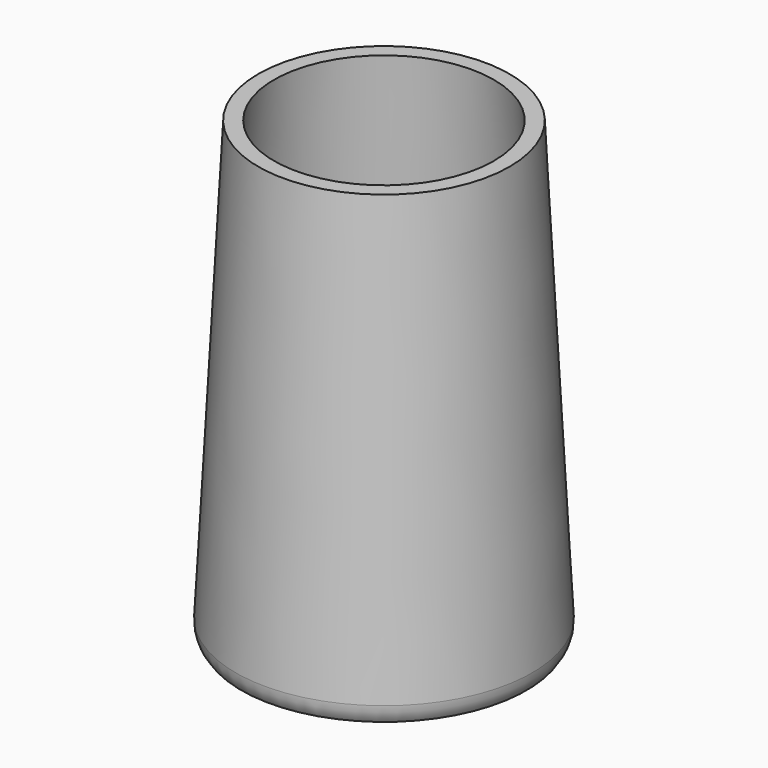
from build123d import *

# Parameters (mm, degrees)
F5_DEPTH = 6.35
F6_T     = -2.54
F7_DEPTH = 25.4
F8_R     = 5.08
F9_R     = 1.27


# Not quite as in the source:
# - a fillet or chamfer that OpenCascade refuses, or shapes differently, is made with other operations: its cross-section is extruded or revolved along the edge and cut away or added


with BuildPart() as f2:
    # F1 (on Front) → F2 (revolve)
    with BuildSketch(Plane.XZ):
        Polygon((-30.1625, 0), (0, 0), (0, 92.075), (-25.4, 92.075), align=None)
    revolve(axis=Axis((0, 0, 46.0375), (0, 0, 1)))

    # F3 (on Front) → F4 (revolve, cut)
    with BuildSketch(Plane.XZ):
        Polygon((0, 92.075), (0, 0), (28.575, 0), (22.225, 92.075), align=None)
    revolve(axis=Axis((0, 0, 46.0375), (0, 0, 1)), mode=Mode.SUBTRACT)

    # F0 (on Top) → F5 (join)
    with BuildSketch(Plane.XY):
        with BuildLine():
            Line((-3.175, -11.3251158636), (-3.175, 23.5998841364))
            ThreePointArc((-3.175, 23.5998841364), (-22.950221268, 6.35), (-14.8542734982, -18.6114404357))
            Line((-14.8542734982, -18.6114404357), (-3.175, -11.3251158636))
        make_face()
        with BuildLine():
            ThreePointArc((23.8125, 0), (17.9253987926, 15.6753065161), (3.175, 23.5998841364))
            Line((3.175, 23.5998841364), (3.175, -11.3251158636))
            Line((3.175, -11.3251158636), (14.8542734982, -18.6114404357))
            ThreePointArc((14.8542734982, -18.6114404357), (21.4563806818, -10.3275788202), (23.8125, 0))
        make_face()
        with BuildLine():
            Line((3.175, -11.3251158636), (3.175, 23.5998841364))
            ThreePointArc((3.175, 23.5998841364), (0, 23.8125), (-3.175, 23.5998841364))
            Line((-3.175, 23.5998841364), (-3.175, -11.3251158636))
            Line((-3.175, -11.3251158636), (-3.175, -23.5998841364))
            ThreePointArc((-3.175, -23.5998841364), (0, -23.8125), (3.175, -23.5998841364))
            Line((3.175, -23.5998841364), (3.175, -11.3251158636))
        make_face()
        with BuildLine():
            Line((3.175, -11.3251158636), (3.175, -23.5998841364))
            ThreePointArc((3.175, -23.5998841364), (9.3533319388, -21.8986378091), (14.8542734982, -18.6114404357))
            Line((14.8542734982, -18.6114404357), (3.175, -11.3251158636))
        make_face()
        with BuildLine():
            ThreePointArc((-14.8542734982, -18.6114404357), (-9.3533319388, -21.8986378091), (-3.175, -23.5998841364))
            Line((-3.175, -23.5998841364), (-3.175, -11.3251158636))
            Line((-3.175, -11.3251158636), (-14.8542734982, -18.6114404357))
        make_face()
        with BuildLine():
            Line((-3.175, 23.5998841364), (-3.175, 28.3980633142))
            ThreePointArc((-3.175, 28.3980633142), (-28.575, 0), (-3.175, -28.3980633142))
            Line((-3.175, -28.3980633142), (-3.175, -23.5998841364))
            ThreePointArc((-3.175, -23.5998841364), (-9.3533319388, -21.8986378091), (-14.8542734982, -18.6114404357))
            ThreePointArc((-14.8542734982, -18.6114404357), (-22.950221268, 6.35), (-3.175, 23.5998841364))
        make_face()
        with BuildLine():
            ThreePointArc((3.175, -28.3980633142), (21.2985474857, -19.05), (28.575, 0))
            ThreePointArc((28.575, 0), (21.2985474857, 19.05), (3.175, 28.3980633142))
            Line((3.175, 28.3980633142), (3.175, 23.5998841364))
            ThreePointArc((3.175, 23.5998841364), (17.9253987926, 15.6753065161), (23.8125, 0))
            ThreePointArc((23.8125, 0), (21.4563806818, -10.3275788202), (14.8542734982, -18.6114404357))
            ThreePointArc((14.8542734982, -18.6114404357), (9.3533319388, -21.8986378091), (3.175, -23.5998841364))
            Line((3.175, -23.5998841364), (3.175, -28.3980633142))
        make_face()
        with BuildLine():
            ThreePointArc((-3.175, -28.3980633142), (0, -28.575), (3.175, -28.3980633142))
            Line((3.175, -28.3980633142), (3.175, -23.5998841364))
            ThreePointArc((3.175, -23.5998841364), (0, -23.8125), (-3.175, -23.5998841364))
            Line((-3.175, -23.5998841364), (-3.175, -28.3980633142))
        make_face()
        with BuildLine():
            Line((3.175, 23.5998841364), (3.175, 28.3980633142))
            ThreePointArc((3.175, 28.3980633142), (0, 28.575), (-3.175, 28.3980633142))
            Line((-3.175, 28.3980633142), (-3.175, 23.5998841364))
            ThreePointArc((-3.175, 23.5998841364), (0, 23.8125), (3.175, 23.5998841364))
        make_face()
    extrude(amount=F5_DEPTH)

    # F6
    f6_openings = [f2.faces().sort_by_distance(p)[0] for p in [
        (0, 0, 0),
    ]]
    offset(amount=F6_T, openings=f6_openings)

    # F0 (on Top) → F7 (cut)
    with BuildSketch(Plane.XY):
        with BuildLine():
            Line((-3.175, -11.3251158636), (-3.175, 23.5998841364))
            ThreePointArc((-3.175, 23.5998841364), (-22.950221268, 6.35), (-14.8542734982, -18.6114404357))
            Line((-14.8542734982, -18.6114404357), (-3.175, -11.3251158636))
        make_face()
        with BuildLine():
            ThreePointArc((23.8125, 0), (17.9253987926, 15.6753065161), (3.175, 23.5998841364))
            Line((3.175, 23.5998841364), (3.175, -11.3251158636))
            Line((3.175, -11.3251158636), (14.8542734982, -18.6114404357))
            ThreePointArc((14.8542734982, -18.6114404357), (21.4563806818, -10.3275788202), (23.8125, 0))
        make_face()
    extrude(amount=F7_DEPTH, mode=Mode.SUBTRACT)

    # F8
    f8_edges = [f2.edges().sort_by_distance(p)[0] for p in [
        (14.854273, -18.61144, 5.08),
        (-14.854273, -18.61144, 5.08),
        (-3.175, -11.325116, 5.08),
        (3.175, -11.325116, 5.08),
        (3.175, 23.599884, 5.08),
        (-3.175, 23.599884, 5.08),
    ]]
    fillet(f8_edges, radius=F8_R)

    # F9
    f9_edges = [f2.edges().sort_by_distance(p)[0] for p in [
        (27.619105, 0, 0),
    ]]
    fillet(f9_edges, radius=F9_R)

    # F10: fillet of radius 5.08 on 1 edges, made by hand

    # F10_s1 → F10_t2 (revolve, cut)
    with BuildSketch(Plane.XZ):
        with BuildLine():
            ThreePointArc((-28.8251126092, 0), (-29.7315388267, 1.6402138976), (-29.9815966442, 3.4974648783))
            Line((-29.9815966442, 3.4974648783), (-30.1625, 0))
            Line((-30.1625, 0), (-28.8251126092, 0))
        make_face()
    revolve(axis=Axis((0, 0, 0), (0, 0, 1)), mode=Mode.SUBTRACT)


solid = f2.part
